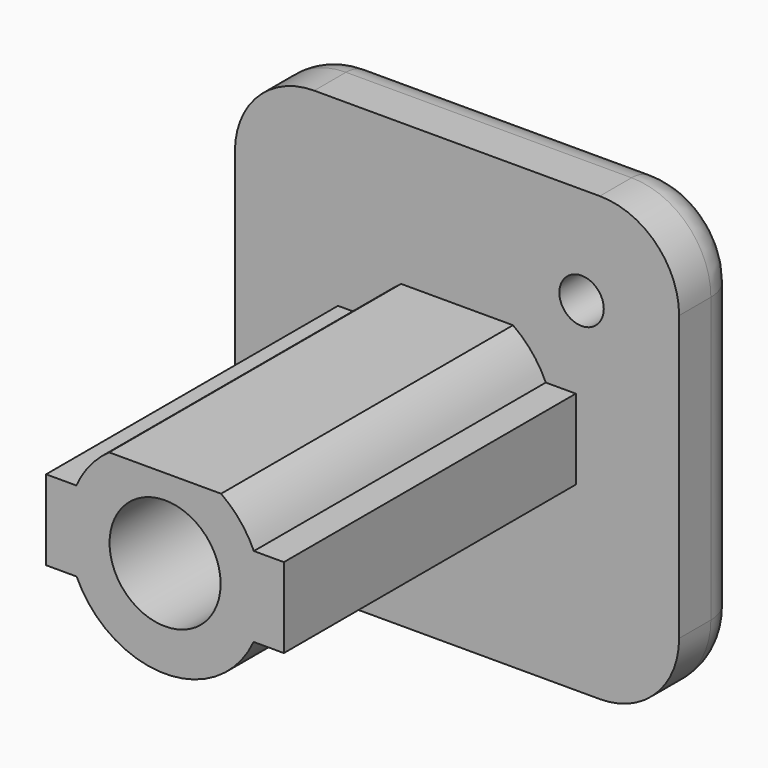
from build123d import *

# Parameters (mm, degrees)
F0_R         = 3.5
F1_DEPTH     = 28
F2_W         = 28
F2_H         = 27.9113203287
F2_R         = 1.4
F3_DEPTH     = 5
F4_R         = 2.5
F5_T1_DEPTH  = 17.5
F5_T4_ANGLE  = 90
F5_T6_ANGLE  = 90
F5_T8_ANGLE  = 90
F5_T10_ANGLE = 90
F0_R_2       = 1.25
F6_DEPTH     = 10


# Not quite as in the source:
# - a fillet or chamfer that OpenCascade refuses, or shapes differently, is made with other operations: its cross-section is extruded or revolved along the edge and cut away or added


with BuildPart() as f1:
    # F0 (on Front) → F1 (new body)
    with BuildSketch(Plane.XZ):
        with BuildLine():
            Line((3.528, 5.0124127732), (-3.528, 5.0124127732))
            ThreePointArc((-3.528, 5.0124127732), (-4.7310778559, 3.8971743778), (-5.5952764673, 2.5027878582))
            Line((-5.5952764673, 2.5027878582), (-7.5016845949, 2.5027878582))
            Line((-7.5016845949, 2.5027878582), (-7.5016845949, -2.5444291532))
            Line((-7.5016845949, -2.5444291532), (-5.5764635831, -2.5444291532))
            ThreePointArc((-5.5764635831, -2.5444291532), (0, -6.1295241095), (5.5764635831, -2.5444291532))
            Line((5.5764635831, -2.5444291532), (7.4870199896, -2.5444291532))
            Line((7.4870199896, -2.5444291532), (7.4870199896, 2.5027878582))
            Line((7.4870199896, 2.5027878582), (5.5952764673, 2.5027878582))
            ThreePointArc((5.5952764673, 2.5027878582), (4.7310778559, 3.8971743778), (3.528, 5.0124127732))
        make_face()
        Circle(F0_R, mode=Mode.SUBTRACT)
    extrude(amount=F1_DEPTH)

    # F2 (on Front) → F3 (join)
    with BuildSketch(Plane.XZ):
        Rectangle(F2_W, F2_H)
        with Locations((-7.7399509028, -7.7685024589)):
            Circle(F2_R, mode=Mode.SUBTRACT)
        with Locations((7.8511200845, 7.7744480222)):
            Circle(F2_R, mode=Mode.SUBTRACT)
    extrude(amount=F3_DEPTH)

    # F4
    f4_edges = [f1.edges().sort_by_distance(p)[0] for p in [
        (14, 0, 0),
        (0, 0, -13.95566),
        (-14, 0, 0),
        (0, 0, 13.95566),
    ]]
    fillet(f4_edges, radius=F4_R)

    # F5: fillet of radius 5 on 4 edges, made by hand

    # F5_s2 → F5_t1 (cut)
    with BuildSketch(Plane.XZ):
        with BuildLine():
            ThreePointArc((-9, 13.9556601644), (-12.5355339059, 12.4911940703), (-14, 8.9556601644))
            Line((-14, 8.9556601644), (-14, 13.9556601644))
            Line((-14, 13.9556601644), (-9, 13.9556601644))
        make_face()
        with BuildLine():
            ThreePointArc((14, 8.9556601644), (12.5355339059, 12.4911940703), (9, 13.9556601644))
            Line((9, 13.9556601644), (14, 13.9556601644))
            Line((14, 13.9556601644), (14, 8.9556601644))
        make_face()
        with BuildLine():
            ThreePointArc((14, -8.9556601644), (12.5355339059, -12.4911940703), (9, -13.9556601644))
            Line((9, -13.9556601644), (14, -13.9556601644))
            Line((14, -13.9556601644), (14, -8.9556601644))
        make_face()
        with BuildLine():
            ThreePointArc((-9, -13.9556601644), (-12.5355339059, -12.4911940703), (-14, -8.9556601644))
            Line((-14, -8.9556601644), (-14, -13.9556601644))
            Line((-14, -13.9556601644), (-9, -13.9556601644))
        make_face()
    extrude(amount=F5_T1_DEPTH, mode=Mode.SUBTRACT)

    # F5_s3 → F5_t4 (revolve, cut)
    with BuildSketch(Plane.YZ.offset(-9)):
        with BuildLine():
            ThreePointArc((0, -11.4556601644), (-0.732233047, -13.2234271173), (-2.5, -13.9556601644))
            Line((-2.5, -13.9556601644), (0, -13.9556601644))
            Line((0, -13.9556601644), (0, -11.4556601644))
        make_face()
    revolve(axis=Axis((-9, 0, -8.9556601644), (0, 1, 0)), revolution_arc=F5_T4_ANGLE, mode=Mode.SUBTRACT)

    # F5_s5 → F5_t6 (revolve, cut)
    with BuildSketch(Plane.XY.offset(-8.9556601644)):
        with BuildLine():
            ThreePointArc((11.5, 0), (13.267766953, -0.732233047), (14, -2.5))
            Line((14, -2.5), (14, 0))
            Line((14, 0), (11.5, 0))
        make_face()
    revolve(axis=Axis((9, 0, -8.9556601644), (0, 1, 0)), revolution_arc=F5_T6_ANGLE, mode=Mode.SUBTRACT)

    # F5_s7 → F5_t8 (revolve, cut)
    with BuildSketch(Plane.YZ.offset(9)):
        with BuildLine():
            ThreePointArc((0, 11.4556601644), (-0.732233047, 13.2234271173), (-2.5, 13.9556601644))
            Line((-2.5, 13.9556601644), (0, 13.9556601644))
            Line((0, 13.9556601644), (0, 11.4556601644))
        make_face()
    revolve(axis=Axis((9, 0, 8.9556601644), (0, 1, 0)), revolution_arc=F5_T8_ANGLE, mode=Mode.SUBTRACT)

    # F5_s9 → F5_t10 (revolve, cut)
    with BuildSketch(Plane.XY.offset(8.9556601644)):
        with BuildLine():
            ThreePointArc((-11.5, 0), (-13.267766953, -0.732233047), (-14, -2.5))
            Line((-14, -2.5), (-14, 0))
            Line((-14, 0), (-11.5, 0))
        make_face()
    revolve(axis=Axis((-9, 0, 8.9556601644), (0, 1, 0)), revolution_arc=F5_T10_ANGLE, mode=Mode.SUBTRACT)

    # F0 (on Front) → F6 (cut)
    with BuildSketch(Plane.XZ):
        Circle(F0_R_2)
    extrude(amount=F6_DEPTH, mode=Mode.SUBTRACT)


solid = f1.part
